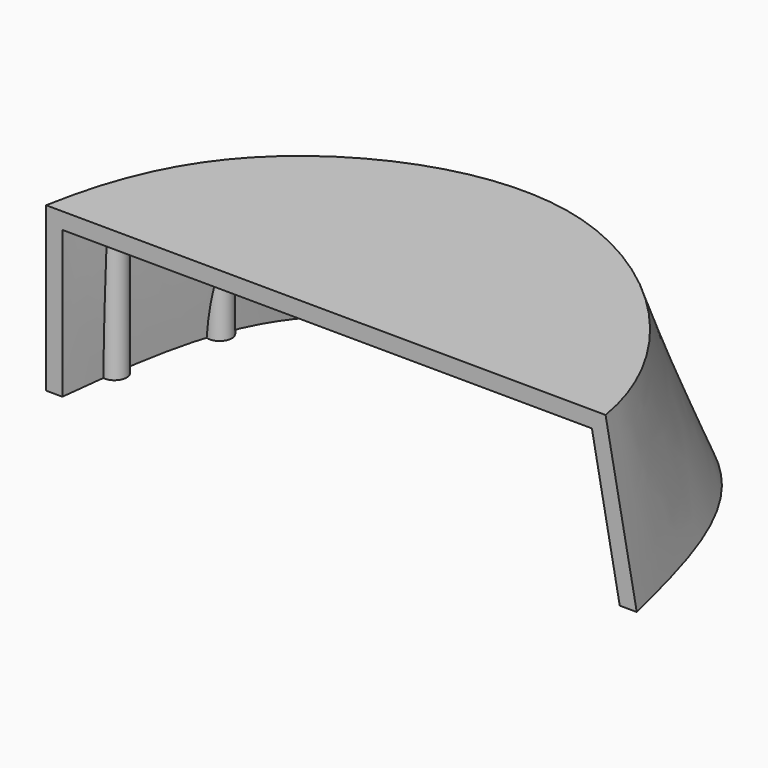
from build123d import *

# Parameters (mm, degrees)
F4_T = -2.54
F5_R = 1.8990139658


with BuildPart() as f3:
    # F2 (on offset) → F3 section 0
    with BuildSketch(Plane.XY.offset(25.4)):
        with BuildLine():
            add(Edge.make_bspline(
                [(-52.1077290177, -31.0851894319), (-49.9430247247, -19.1282802679), (-41.2628958229, 0.046348237), (2.4314136161, 17.1871001704), (32.7174059217, -14.4476079542), (35.4601876655, -31.7134802652)],
                knots=[0, 0, 0, 0, 0.2950998903, 0.6209843962, 1, 1, 1, 1], degree=3))
            Line((-52.1077290177, -31.0851894319), (35.4601876655, -31.7134802652))
        make_face()
    # F0 (on Top) → F3 section 1
    with BuildSketch(Plane.XY):
        with BuildLine():
            add(Edge.make_bspline(
                [(-52.1077290177, -31.0851894319), (-50.4575478756, -16.2377927152), (-47.1497979531, 13.5234705089), (1.3002766568, 19.8238403002), (31.8592244074, 2.7564081899), (37.4932082867, -20.1464899268), (40.3472483158, -31.7485444248)],
                knots=[0, 0, 0, 0, 0.2617854816, 0.5247429415, 0.7592462637, 1, 1, 1, 1], degree=3))
            Line((-52.1077290177, -31.0851894319), (40.3472483158, -31.7485444248))
        make_face()
    loft()

    # F4
    f4_openings = [f3.faces().sort_by_distance(p)[0] for p in [
        (-7.09095, -31.40818, 12.585078),
        (-7.452568, -10.520287, 0),
    ]]
    offset(amount=F4_T, openings=f4_openings)


with BuildPart() as f6:
    # F5 (on face) → F6 (new body, up to the next surface of F3)
    with BuildSketch(Plane(origin=(0, 0, 0), x_dir=(1, 0, 0), z_dir=(0, 0, -1))):
        with Locations((-48.5022947899, 22.2912294291)):
            Circle(F5_R)
    extrude(until=Until.NEXT, target=f3.part, dir=(0, 0, 1))


with BuildPart() as f6b:
    # F5 (on face) → F6, piece 2 (new body, up to the next surface of F3)
    with BuildSketch(Plane(origin=(0, 0, 0), x_dir=(1, 0, 0), z_dir=(0, 0, -1))):
        with Locations((-44.9746544949, 6.2390208126)):
            Circle(F5_R)
    extrude(until=Until.NEXT, target=f3.part, dir=(0, 0, 1))


solid = Compound([f3.part, f6.part, f6b.part])
